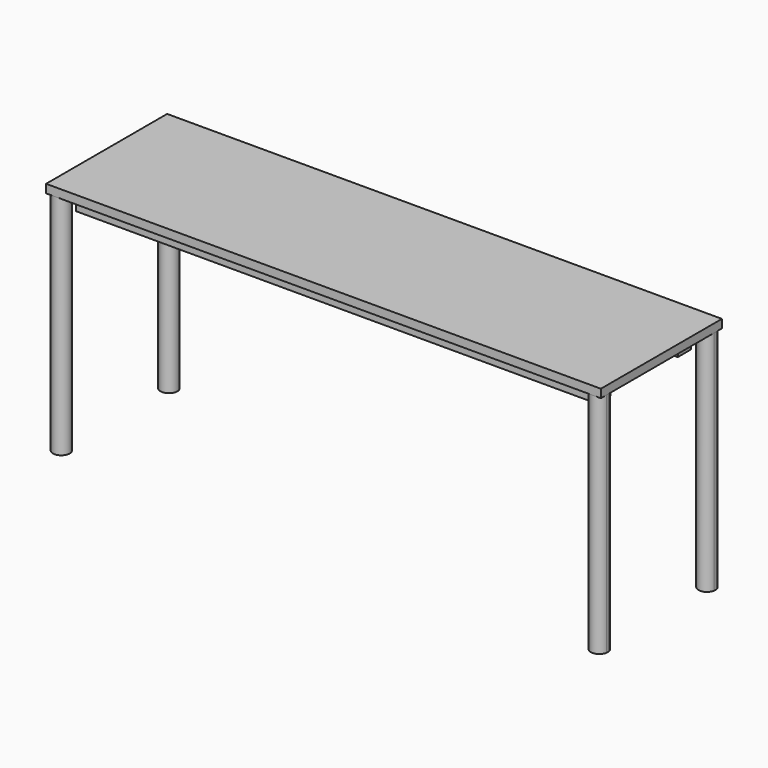
from build123d import *

# Parameters (mm, degrees)
F0_W     = 1676.4
F0_H     = 457.2
F1_DEPTH = 25.4
F2_R     = 25.4
F3_DEPTH = 685.8
F5_DEPTH = 50.8


with BuildPart() as f1:
    # F0 (on Top) → F1 (new body)
    with BuildSketch(Plane.XY):
        with Locations((-842.7907367021, -333.0861411702)):
            Rectangle(F0_W, F0_H)
    extrude(amount=F1_DEPTH)

    # F4 (on face) → F5 (join)
    with BuildSketch(Plane.XY):
        Polygon((-1629.9590991974, -461.9765826102), (-1629.9590991974, -512.7765826102), (-1604.5590991974, -512.7765826102), (-1579.1590991974, -512.7765826102), (-55.1590991974, -512.7765826102), (-55.1590991974, -461.9765826102), (-1579.1590991974, -461.9765826102), (-1604.5590991974, -461.9765826102), align=None)
        Polygon((-1579.1590991974, -207.9765826102), (-55.1590991974, -207.9765826102), (-55.1590991974, -157.1765826102), (-1579.1590991974, -157.1765826102), (-1604.5590991974, -157.1765826102), (-1629.9590991974, -157.1765826102), (-1629.9590991974, -207.9765826102), (-1604.5590991974, -207.9765826102), align=None)
    extrude(amount=-F5_DEPTH)


with BuildPart() as f3:
    # F2 (on face) → F3 (new body)
    with BuildSketch(Plane.XY):
        with Locations((-1655.2361249924, -536.1693501472)):
            Circle(F2_R)
    extrude(amount=-F3_DEPTH)


with BuildPart() as f3b:
    # F2 (on face) → F3, piece 2 (new body)
    with BuildSketch(Plane.XY):
        with BuildLine():
            ThreePointArc((-1657.6690951571, -104.4861411702), (-1672.3148040662, -148.5703799353), (-1629.8361249924, -129.7693501472))
            ThreePointArc((-1629.8361249924, -129.7693501472), (-1636.4350952043, -112.6906710734), (-1652.8031548277, -104.4861411702))
            Line((-1652.8031548277, -104.4861411702), (-1657.6690951571, -104.4861411702))
        make_face()
    extrude(amount=-F3_DEPTH)


with BuildPart() as f3c:
    # F2 (on face) → F3, piece 3 (new body)
    with BuildSketch(Plane.XY):
        with BuildLine():
            Line((-27.2031548277, -104.4861411702), (-32.0690951571, -104.4861411702))
            ThreePointArc((-32.0690951571, -104.4861411702), (-48.2259100492, -147.0777264877), (-4.5907367021, -133.9988330221))
            Line((-4.5907367021, -133.9988330221), (-4.5907367021, -125.5398672724))
            ThreePointArc((-4.5907367021, -125.5398672724), (-12.3277486519, -111.1795650904), (-27.2031548277, -104.4861411702))
        make_face()
    extrude(amount=-F3_DEPTH)


with BuildPart() as f3d:
    # F2 (on face) → F3, piece 4 (new body)
    with BuildSketch(Plane.XY):
        with BuildLine():
            Line((-4.5907367021, -540.3988330221), (-4.5907367021, -531.9398672724))
            ThreePointArc((-4.5907367021, -531.9398672724), (-55.0361249924, -536.1693501472), (-4.5907367021, -540.3988330221))
        make_face()
    extrude(amount=-F3_DEPTH)


solid = Compound([f1.part, f3.part, f3b.part, f3c.part, f3d.part])
